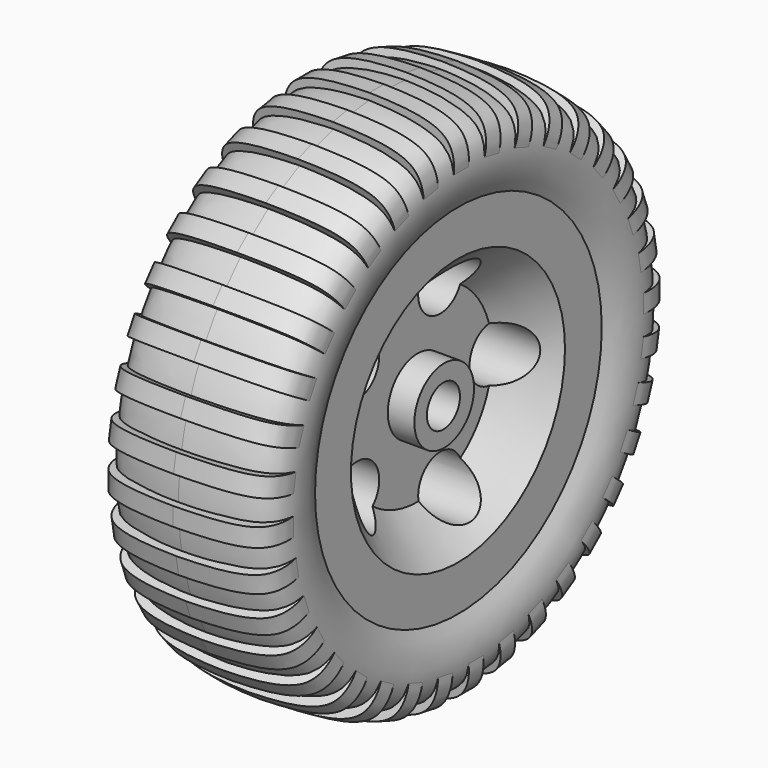
from build123d import *

# Parameters (mm, degrees)
F3_R      = 2.25
F4_DEPTH  = 25
F5_R      = 3
F6_DEPTH  = 25
F10_DEPTH = 2
F11_COUNT = 36


# Not quite as in the source:
# - a feature names something its author has since deleted; it is built from what else it names


with BuildPart() as f2:
    # F0 (on Top) → F2 (revolve)
    with BuildSketch(Plane.XY):
        Polygon((0, -5), (0, 0), (-3, 0), (-3, -2), (-11, -2), (-13, 0), (-16, 0), (-16, -5), (-11.6092312851, -9.3907687149), (-11.6092312851, -15.5), (-14.5, -15.5), (-14.5, -19.5), (-1.5, -19.5), (-1.5, -15.5), (-4.3907687149, -15.5), (-4.3907687149, -9.3907687149), align=None)
    revolve(axis=Axis((0, -19.5563957095, 0), (1, 0, 0)))

    # F3 (on Right) → F4 (cut)
    with BuildSketch(Plane.YZ):
        with Locations((-19.6564700454, 0)):
            Circle(F3_R)
    extrude(amount=-F4_DEPTH, mode=Mode.SUBTRACT)

    # F5 (on Right) → F6 (cut)
    with BuildSketch(Plane.YZ):
        with Locations((-9.4930212945, 0)):
            Circle(F5_R)
        with Locations((-27.7767175346, 5.9407330283)):
            Circle(F5_R)
        with Locations((-27.7767175346, -5.9407330283)):
            Circle(F5_R)
        with Locations((-16.4767718182, -9.6123079579)):
            Circle(F5_R)
        with Locations((-16.4767718182, 9.6123079579)):
            Circle(F5_R)
    extrude(amount=-F6_DEPTH, mode=Mode.SUBTRACT)


with BuildPart() as f8:
    # F7 (on Top) → F8 (revolve)
    with BuildSketch(Plane.XY):
        with BuildLine():
            Line((-3, 0), (0, 0))
            add(Edge.make_bspline(
                [(0, 0), (0.3545977923, 0.6547178688), (0.8945018578, 1.7128395264), (1.1895318368, 3.1212979751), (1.3232356914, 4.592825874), (0.4536476467, 7.8977585567), (-5.0962997451, 8.5160154849), (-8, 8.569046855)],
                knots=[0, 0, 0, 0, 0.169898326, 0.3112196225, 0.4560927849, 0.6542283688, 1, 1, 1, 1], degree=3))
            add(Edge.make_bspline(
                [(-16, 0), (-16.3545977923, 0.6547178688), (-16.8945018578, 1.7128395264), (-17.1895318368, 3.1212979751), (-17.3232356914, 4.592825874), (-16.4536476467, 7.8977585567), (-10.9037002549, 8.5160154849), (-8, 8.569046855)],
                knots=[0, 0, 0, 0, 0.169898326, 0.3112196225, 0.4560927849, 0.6542283688, 1, 1, 1, 1], degree=3))
            Line((-16, 0), (-13.0105381832, 0))
            Line((-13.0105381832, 0), (-11.0105381832, -2))
            Line((-11.0105381832, -2), (-3, -2))
            Line((-3, -2), (-3, 0))
        make_face()
    revolve(axis=Axis((-5.8021252044, -19.5, 0), (1, 0, 0)))


with BuildPart() as f10:
    # F9 (on Top) → F10 (new body)
    with BuildSketch(Plane.XY):
        with BuildLine():
            add(Edge.make_bspline(
                [(1.2326572663, 4.1587883827), (1.1446242269, 4.8954475745), (0.3873066334, 7.4672960651), (-5.0707449288, 7.7533862509), (-7.968747437, 7.8063135609)],
                knots=[0.466920007, 0.466920007, 0.466920007, 0.466920007, 0.6549068546, 1, 1, 1, 1], degree=3))
            add(Edge.make_bspline(
                [(1.2326572663, 4.1587883827), (1.272711411, 4.5052809487), (1.313050881, 5.4970566833), (0.4933204745, 8.7171360951), (-5.0707449288, 9.0087831209), (-7.968747437, 9.0617104308)],
                knots=[0.3438842769, 0.3438842769, 0.3438842769, 0.3438842769, 0.4565657886, 0.6549068546, 1, 1, 1, 1], degree=3))
            add(Edge.make_bspline(
                [(-17.1701521403, 4.1587883827), (-17.210206285, 4.5052809487), (-17.250545755, 5.4970566833), (-16.4308153485, 8.7171360951), (-10.8667499452, 9.0087831209), (-7.968747437, 9.0617104308)],
                knots=[0.3438842769, 0.3438842769, 0.3438842769, 0.3438842769, 0.4565657886, 0.6549068546, 1, 1, 1, 1], degree=3))
            add(Edge.make_bspline(
                [(-17.1701521403, 4.1587883827), (-17.0821191009, 4.8954475745), (-16.3248015074, 7.4672960651), (-10.8667499452, 7.7533862509), (-7.968747437, 7.8063135609)],
                knots=[0.466920007, 0.466920007, 0.466920007, 0.466920007, 0.6549068546, 1, 1, 1, 1], degree=3))
        make_face()
    extrude(amount=F10_DEPTH)


with BuildPart() as f11_1:
    # F11: instance of F10
    add(f10.part.rotate(Axis((-1.5, -19.6564700454, 0), (1, 0, 0)), 1 * 360 / F11_COUNT))


with BuildPart() as f11_2:
    # F11: instance of F10
    add(f10.part.rotate(Axis((-1.5, -19.6564700454, 0), (1, 0, 0)), 2 * 360 / F11_COUNT))


with BuildPart() as f11_3:
    # F11: instance of F10
    add(f10.part.rotate(Axis((-1.5, -19.6564700454, 0), (1, 0, 0)), 3 * 360 / F11_COUNT))


with BuildPart() as f11_4:
    # F11: instance of F10
    add(f10.part.rotate(Axis((-1.5, -19.6564700454, 0), (1, 0, 0)), 4 * 360 / F11_COUNT))


with BuildPart() as f11_5:
    # F11: instance of F10
    add(f10.part.rotate(Axis((-1.5, -19.6564700454, 0), (1, 0, 0)), 5 * 360 / F11_COUNT))


with BuildPart() as f11_6:
    # F11: instance of F10
    add(f10.part.rotate(Axis((-1.5, -19.6564700454, 0), (1, 0, 0)), 6 * 360 / F11_COUNT))


with BuildPart() as f11_7:
    # F11: instance of F10
    add(f10.part.rotate(Axis((-1.5, -19.6564700454, 0), (1, 0, 0)), 7 * 360 / F11_COUNT))


with BuildPart() as f11_8:
    # F11: instance of F10
    add(f10.part.rotate(Axis((-1.5, -19.6564700454, 0), (1, 0, 0)), 8 * 360 / F11_COUNT))


with BuildPart() as f11_9:
    # F11: instance of F10
    add(f10.part.rotate(Axis((-1.5, -19.6564700454, 0), (1, 0, 0)), 9 * 360 / F11_COUNT))


with BuildPart() as f11_10:
    # F11: instance of F10
    add(f10.part.rotate(Axis((-1.5, -19.6564700454, 0), (1, 0, 0)), 10 * 360 / F11_COUNT))


with BuildPart() as f11_11:
    # F11: instance of F10
    add(f10.part.rotate(Axis((-1.5, -19.6564700454, 0), (1, 0, 0)), 11 * 360 / F11_COUNT))


with BuildPart() as f11_12:
    # F11: instance of F10
    add(f10.part.rotate(Axis((-1.5, -19.6564700454, 0), (1, 0, 0)), 12 * 360 / F11_COUNT))


with BuildPart() as f11_13:
    # F11: instance of F10
    add(f10.part.rotate(Axis((-1.5, -19.6564700454, 0), (1, 0, 0)), 13 * 360 / F11_COUNT))


with BuildPart() as f11_14:
    # F11: instance of F10
    add(f10.part.rotate(Axis((-1.5, -19.6564700454, 0), (1, 0, 0)), 14 * 360 / F11_COUNT))


with BuildPart() as f11_15:
    # F11: instance of F10
    add(f10.part.rotate(Axis((-1.5, -19.6564700454, 0), (1, 0, 0)), 15 * 360 / F11_COUNT))


with BuildPart() as f11_16:
    # F11: instance of F10
    add(f10.part.rotate(Axis((-1.5, -19.6564700454, 0), (1, 0, 0)), 16 * 360 / F11_COUNT))


with BuildPart() as f11_17:
    # F11: instance of F10
    add(f10.part.rotate(Axis((-1.5, -19.6564700454, 0), (1, 0, 0)), 17 * 360 / F11_COUNT))


with BuildPart() as f11_18:
    # F11: instance of F10
    add(f10.part.rotate(Axis((-1.5, -19.6564700454, 0), (1, 0, 0)), 18 * 360 / F11_COUNT))


with BuildPart() as f11_19:
    # F11: instance of F10
    add(f10.part.rotate(Axis((-1.5, -19.6564700454, 0), (1, 0, 0)), 19 * 360 / F11_COUNT))


with BuildPart() as f11_20:
    # F11: instance of F10
    add(f10.part.rotate(Axis((-1.5, -19.6564700454, 0), (1, 0, 0)), 20 * 360 / F11_COUNT))


with BuildPart() as f11_21:
    # F11: instance of F10
    add(f10.part.rotate(Axis((-1.5, -19.6564700454, 0), (1, 0, 0)), 21 * 360 / F11_COUNT))


with BuildPart() as f11_22:
    # F11: instance of F10
    add(f10.part.rotate(Axis((-1.5, -19.6564700454, 0), (1, 0, 0)), 22 * 360 / F11_COUNT))


with BuildPart() as f11_23:
    # F11: instance of F10
    add(f10.part.rotate(Axis((-1.5, -19.6564700454, 0), (1, 0, 0)), 23 * 360 / F11_COUNT))


with BuildPart() as f11_24:
    # F11: instance of F10
    add(f10.part.rotate(Axis((-1.5, -19.6564700454, 0), (1, 0, 0)), 24 * 360 / F11_COUNT))


with BuildPart() as f11_25:
    # F11: instance of F10
    add(f10.part.rotate(Axis((-1.5, -19.6564700454, 0), (1, 0, 0)), 25 * 360 / F11_COUNT))


with BuildPart() as f11_26:
    # F11: instance of F10
    add(f10.part.rotate(Axis((-1.5, -19.6564700454, 0), (1, 0, 0)), 26 * 360 / F11_COUNT))


with BuildPart() as f11_27:
    # F11: instance of F10
    add(f10.part.rotate(Axis((-1.5, -19.6564700454, 0), (1, 0, 0)), 27 * 360 / F11_COUNT))


with BuildPart() as f11_28:
    # F11: instance of F10
    add(f10.part.rotate(Axis((-1.5, -19.6564700454, 0), (1, 0, 0)), 28 * 360 / F11_COUNT))


with BuildPart() as f11_29:
    # F11: instance of F10
    add(f10.part.rotate(Axis((-1.5, -19.6564700454, 0), (1, 0, 0)), 29 * 360 / F11_COUNT))


with BuildPart() as f11_30:
    # F11: instance of F10
    add(f10.part.rotate(Axis((-1.5, -19.6564700454, 0), (1, 0, 0)), 30 * 360 / F11_COUNT))


with BuildPart() as f11_31:
    # F11: instance of F10
    add(f10.part.rotate(Axis((-1.5, -19.6564700454, 0), (1, 0, 0)), 31 * 360 / F11_COUNT))


with BuildPart() as f11_32:
    # F11: instance of F10
    add(f10.part.rotate(Axis((-1.5, -19.6564700454, 0), (1, 0, 0)), 32 * 360 / F11_COUNT))


with BuildPart() as f11_33:
    # F11: instance of F10
    add(f10.part.rotate(Axis((-1.5, -19.6564700454, 0), (1, 0, 0)), 33 * 360 / F11_COUNT))


with BuildPart() as f11_34:
    # F11: instance of F10
    add(f10.part.rotate(Axis((-1.5, -19.6564700454, 0), (1, 0, 0)), 34 * 360 / F11_COUNT))


with BuildPart() as f11_35:
    # F11: instance of F10
    add(f10.part.rotate(Axis((-1.5, -19.6564700454, 0), (1, 0, 0)), 35 * 360 / F11_COUNT))


solid = Compound([f2.part, f8.part, f10.part, f11_1.part, f11_2.part, f11_3.part, f11_4.part, f11_5.part, f11_6.part, f11_7.part, f11_8.part, f11_9.part, f11_10.part, f11_11.part, f11_12.part, f11_13.part, f11_14.part, f11_15.part, f11_16.part, f11_17.part, f11_18.part, f11_19.part, f11_20.part, f11_21.part, f11_22.part, f11_23.part, f11_24.part, f11_25.part, f11_26.part, f11_27.part, f11_28.part, f11_29.part, f11_30.part, f11_31.part, f11_32.part, f11_33.part, f11_34.part, f11_35.part])
